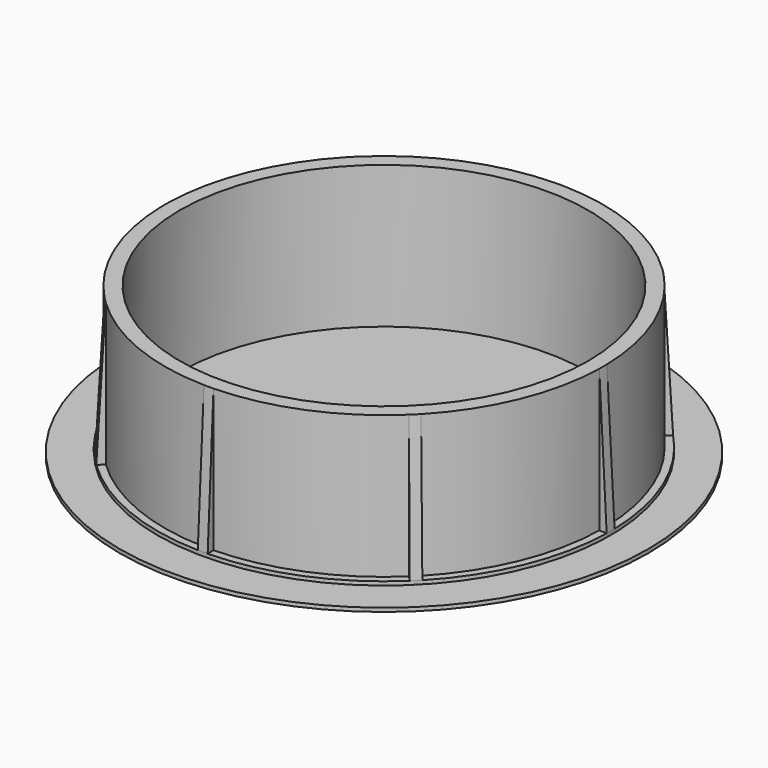
from build123d import *

# Parameters (mm, degrees)
F2_ANGLE_BACK = 1.25
F2_ANGLE      = 2.5
F3_COUNT      = 8


# Not quite as in the source:
# - a feature names something its author has since deleted; it is built from what else it names


with BuildPart() as f1:
    # F0 (on Front) → F1 (revolve)
    with BuildSketch(Plane.XZ):
        Polygon((0, 0.5), (-30.25, 0.5), (-35.25, 0.5), (-35.25, 0), (0, 0), align=None)
        Polygon((-29.25, 1), (-30.25, 1), (-30.25, 0.5), (0, 0.5), (0, 1), (-27.25, 1), (-27.25, 20), (-29.25, 20), align=None)
    revolve(axis=Axis((0, 0, 0.5), (0, 0, -1)))

    # F0 (on Front) → F2 (revolve)
    with BuildSketch(Plane.XZ, mode=Mode.PRIVATE) as f2_sk:
        Polygon((-29.25, 20), (-30.25, 1), (-29.25, 1), align=None)
    revolve(f2_sk.sketch.rotate(Axis((0, 0, 0.5), (0, 0, -1)), -F2_ANGLE_BACK), axis=Axis((0, 0, 0.5), (0, 0, -1)), revolution_arc=F2_ANGLE)

    # F3: F1 ×8 about axis
    f3_axis = Axis((0, 0, 0.5), (0, 0, -1))


with BuildPart() as f1_1:
    add(f1.part)
    for i in range(1, F3_COUNT):
        add(f1.part.rotate(f3_axis, i * 360 / F3_COUNT))


solid = f1_1.part
